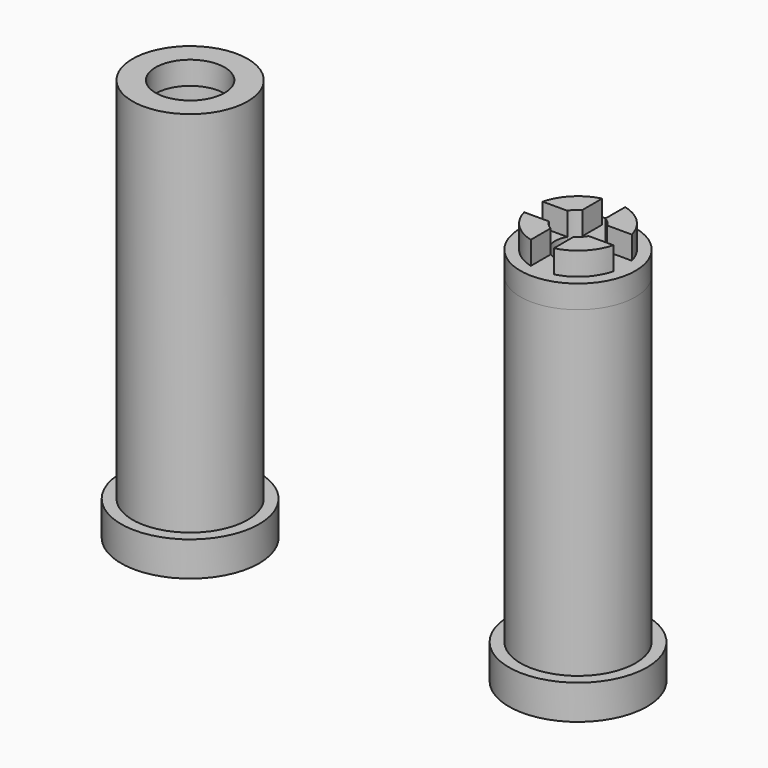
from build123d import *

# Parameters (mm, degrees)
F0_R      = 6
F0_R_2    = 5
F0_R_3    = 2
F1_DEPTH  = 3
F2_R      = 5
F2_R_2    = 2
F3_DEPTH  = 28
F4_R      = 3
F4_R_2    = 2
F5_DEPTH  = 2
F6_R      = 4
F6_R_2    = 3
F6_R_3    = 2
F7_DEPTH  = 2
F8_W      = 2
F8_H      = 3
F8_H_2    = 2
F8_W_2    = 3
F9_DEPTH  = 4
F10_R     = 5
F10_R_2   = 2
F11_DEPTH = 28
F12_R     = 5
F12_R_2   = 4
F13_DEPTH = 2
F14_R     = 5
F14_R_2   = 4
F14_R_3   = 3
F9_FACE_R = 5
F15_DEPTH = 2


with BuildPart() as f1:
    # F0 (on Top) → F1 (new body)
    with BuildSketch(Plane.XY):
        with Locations((-17.0216653496, 0)):
            Circle(F0_R)
        with Locations((-17.0216653496, 0)):
            Circle(F0_R_2, mode=Mode.SUBTRACT)
        with Locations((-17.0216653496, 0)):
            Circle(F0_R_2)
        with Locations((-17.0216653496, 0)):
            Circle(F0_R_3, mode=Mode.SUBTRACT)
    extrude(amount=F1_DEPTH)

    # F10 (on face) → F11 (join)
    with BuildSketch(Plane.XY.offset(3)):
        with Locations((-17.0216653496, 0)):
            Circle(F10_R)
        with Locations((-17.0216653496, 0)):
            Circle(F10_R_2, mode=Mode.SUBTRACT)
    extrude(amount=F11_DEPTH)

    # F12 (on face) → F13 (join)
    with BuildSketch(Plane.XY.offset(31)):
        with Locations((-17.0216653496, 0)):
            Circle(F12_R)
        with Locations((-17.0216653496, 0)):
            Circle(F12_R_2, mode=Mode.SUBTRACT)
    extrude(amount=F13_DEPTH)

    # F14 (on face) + F9_face (on face) → F15 (join)
    with BuildSketch(Plane.XY.offset(33)):
        with Locations((-17.0216653496, 0)):
            Circle(F14_R)
        with Locations((-17.0216653496, 0)):
            Circle(F14_R_2, mode=Mode.SUBTRACT)
        with Locations((-17.0216653496, 0)):
            Circle(F14_R_2)
        with Locations((-17.0216653496, 0)):
            Circle(F14_R_3, mode=Mode.SUBTRACT)
    with BuildSketch(Plane(origin=(16.6711099446, 0, 31), x_dir=(1, 0, 0), z_dir=(0, 0, 1))):
        Circle(F9_FACE_R)
        with BuildLine():
            ThreePointArc((2, 0), (1.9318516526, -0.5176380902), (1.7320508076, -1))
            Line((1.7320508076, -1), (2.8284271247, -1))
            ThreePointArc((2.8284271247, -1), (2.1213203436, -2.1213203436), (1, -2.8284271247))
            Line((1, -2.8284271247), (1, -1.7320508076))
            ThreePointArc((1, -1.7320508076), (0, -2), (-1, -1.7320508076))
            Line((-1, -1.7320508076), (-1, -2.8284271247))
            ThreePointArc((-1, -2.8284271247), (-2.1213203436, -2.1213203436), (-2.8284271247, -1))
            Line((-2.8284271247, -1), (-1.7320508076, -1))
            ThreePointArc((-1.7320508076, -1), (-2, 0), (-1.7320508076, 1))
            Line((-1.7320508076, 1), (-2.8284271247, 1))
            ThreePointArc((-2.8284271247, 1), (-2.1213203436, 2.1213203436), (-1, 2.8284271247))
            Line((-1, 2.8284271247), (-1, 1.7320508076))
            ThreePointArc((-1, 1.7320508076), (0, 2), (1, 1.7320508076))
            Line((1, 1.7320508076), (1, 2.8284271247))
            ThreePointArc((1, 2.8284271247), (2.1213203436, 2.1213203436), (2.8284271247, 1))
            Line((2.8284271247, 1), (1.7320508076, 1))
            ThreePointArc((1.7320508076, 1), (1.9318516526, 0.5176380902), (2, 0))
        make_face(mode=Mode.SUBTRACT)
    extrude(amount=F15_DEPTH)


with BuildPart() as f1b:
    # F0 (on Top) → F1, piece 2 (new body)
    with BuildSketch(Plane.XY):
        with Locations((16.6711099446, 0)):
            Circle(F0_R)
        with Locations((16.6711099446, 0)):
            Circle(F0_R_2, mode=Mode.SUBTRACT)
        with Locations((16.6711099446, 0)):
            Circle(F0_R_2)
        with Locations((16.6711099446, 0)):
            Circle(F0_R_3, mode=Mode.SUBTRACT)
    extrude(amount=F1_DEPTH)

    # F2 (on face) → F3 (join)
    with BuildSketch(Plane.XY.offset(3)):
        with Locations((16.6711099446, 0)):
            Circle(F2_R)
        with Locations((16.6711099446, 0)):
            Circle(F2_R_2, mode=Mode.SUBTRACT)
    extrude(amount=F3_DEPTH)

    # F4 (on face) → F5 (join)
    with BuildSketch(Plane.XY.offset(31)):
        with Locations((16.6711099446, 0)):
            Circle(F4_R)
        with Locations((16.6711099446, 0)):
            Circle(F4_R_2, mode=Mode.SUBTRACT)
    extrude(amount=F5_DEPTH)

    # F6 (on face) → F7 (join)
    with BuildSketch(Plane.XY.offset(33)):
        with Locations((16.6711099446, 0)):
            Circle(F6_R)
        with Locations((16.6711099446, 0)):
            Circle(F6_R_2, mode=Mode.SUBTRACT)
        with Locations((16.6711099446, 0)):
            Circle(F6_R_2)
        with Locations((16.6711099446, 0)):
            Circle(F6_R_3, mode=Mode.SUBTRACT)
    extrude(amount=F7_DEPTH)

    # F8 (on face) → F9 (cut)
    with BuildSketch(Plane.XY.offset(35)):
        with Locations((16.6711099446, -2.5)):
            Rectangle(F8_W, F8_H)
        with Locations((16.6711099446, 0)):
            Rectangle(F8_W, F8_H_2)
        with Locations((19.1711099446, 0)):
            Rectangle(F8_W_2, F8_H_2)
        with Locations((16.6711099446, 2.5)):
            Rectangle(F8_W, F8_H)
        with Locations((14.1711099446, 0)):
            Rectangle(F8_W_2, F8_H_2)
    extrude(amount=-F9_DEPTH, mode=Mode.SUBTRACT)


solid = Compound([f1.part, f1b.part])
